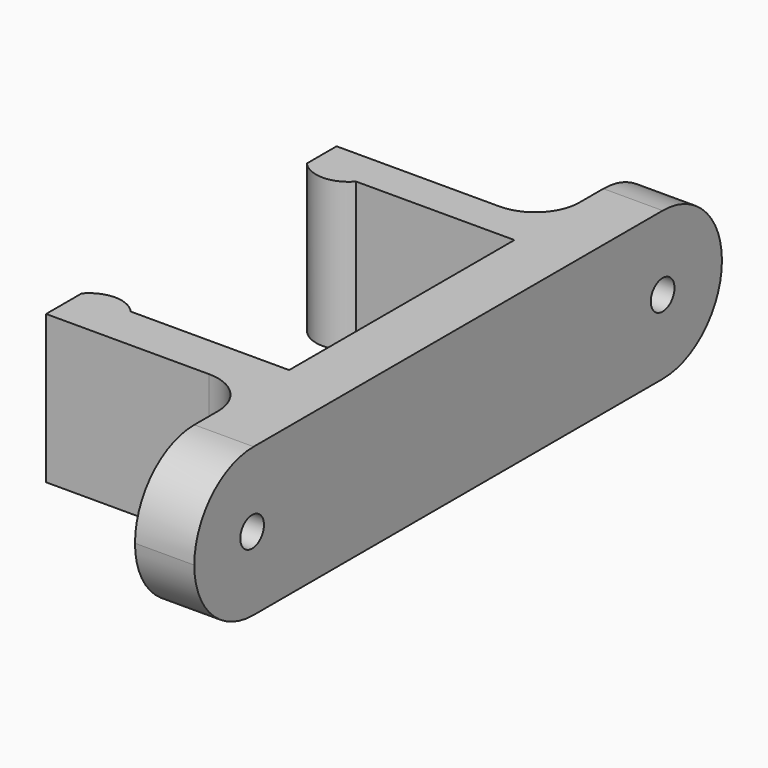
from build123d import *

# Parameters (mm, degrees)
F1_DEPTH = 10
F3_D     = 2
F4_R     = 4.99999
F5_R     = 3


# Not quite as in the source:
# - a fillet or chamfer is up to 0.001 mm smaller than in the source, because OpenCascade refuses the exact size
# - a feature names something its author has since deleted; it is built from what else it names


with BuildPart() as f1:
    # F0 (on Top) → F1 (new body)
    with BuildSketch(Plane.XY):
        with BuildLine():
            Line((-12.6909215784, 9.75), (-16, 9.75))
            ThreePointArc((-16, 9.75), (-14.3454607892, 9), (-12.6909215784, 9.75))
        make_face()
        Polygon((2, -22.25), (2, -12.25), (2, 12.25), (2, 22.25), (-2, 22.25), (-2, 12.25), (-16, 12.25), (-16, 9.75), (-12.6909215784, 9.75), (-2, 9.75), (-2, -9.25), (-12.6909215784, -9.25), (-16, -9.25), (-16, -12.25), (-2, -12.25), (-2, -22.25), align=None)
        with BuildLine():
            ThreePointArc((-12.6909215784, -9.25), (-14.3454607892, -8.5), (-16, -9.25))
            Line((-16, -9.25), (-12.6909215784, -9.25))
        make_face()
    extrude(amount=F1_DEPTH)

    # F3 (through all)
    with Locations(Plane(origin=(-2, 0, 0), x_dir=(0, -1, 0), z_dir=(-1, 0, 0))):
        with Locations((-17.25, 5), (17.3738710582, 5)):
            Hole(F3_D / 2)

    # F4 (radius 5 in the source; OpenCascade refuses exactly that, so slightly less here)
    f4_edges = [f1.edges().sort_by_distance(p)[0] for p in [
        (0, 22.25, 10),
        (0, -22.25, 10),
        (0, -22.25, 0),
        (0, 22.25, 0),
    ]]
    fillet(f4_edges, radius=F4_R)

    # F5
    f5_edges = [f1.edges().sort_by_distance(p)[0] for p in [
        (-2, 12.25, 5),
        (-2, -12.25, 5),
    ]]
    fillet(f5_edges, radius=F5_R)


solid = f1.part
